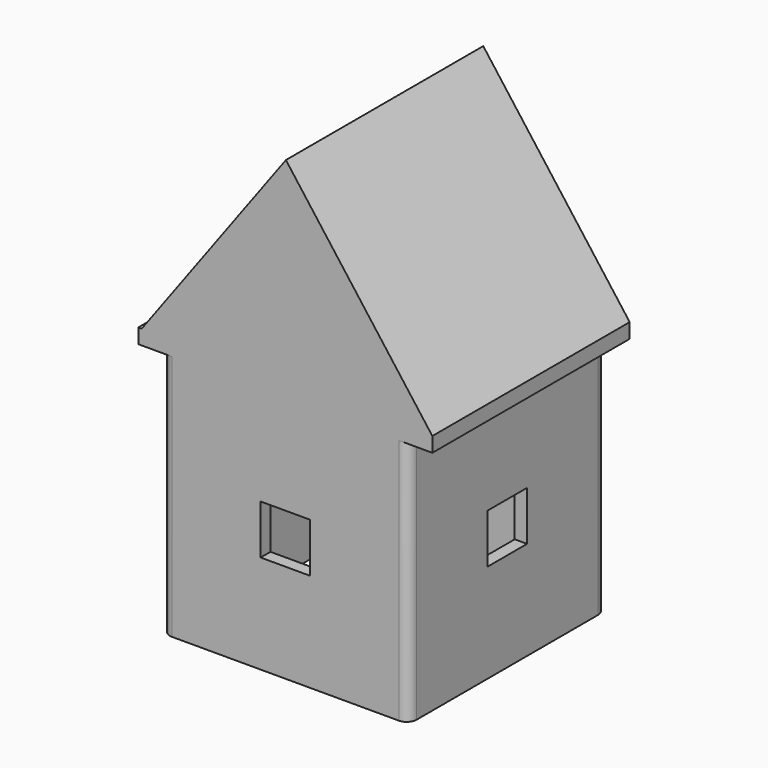
from build123d import *

# Parameters (mm, degrees)
F0_W      = 127
F0_H      = 127
F0_W_2    = 114.3
F0_H_2    = 114.3
F1_DEPTH  = 127
F2_W      = 25.4
F2_H      = 25.4
F3_DEPTH  = 6.35
F6_COUNT  = 4
F7_R      = 5.08
F9_DEPTH  = 7.62
F11_DEPTH = 127


with BuildPart() as f1:
    # F0 (on Top) → F1 (new body)
    with BuildSketch(Plane.XY):
        with Locations((-0.4615932703, 33.8642211668)):
            Rectangle(F0_W, F0_H)
        with Locations((-0.4615932703, 33.8642211668)):
            Rectangle(F0_W_2, F0_H_2, mode=Mode.SUBTRACT)
    extrude(amount=F1_DEPTH)

    # F2 (on face) → F3 (cut, through all)
    with BuildSketch(Plane.YZ.offset(63.0384067297)):
        with Locations((33.8642211668, 63.5)):
            Rectangle(F2_W, F2_H)
    f3 = extrude(amount=-F3_DEPTH, mode=Mode.SUBTRACT)

    # F6: F3 ×4 about axis
    f6_axis = Axis((-0.4615932703, 33.8642211668, 78.3742320016), (0, 0, -1))
    for i in range(1, F6_COUNT):
        add(f3.rotate(f6_axis, i * 360 / F6_COUNT), mode=Mode.SUBTRACT)

    # F7
    f7_edges = [f1.edges().sort_by_distance(p)[0] for p in [
        (-63.961593, -29.635779, 63.5),
        (63.038407, -29.635779, 63.5),
        (-63.961593, 97.364221, 63.5),
        (56.688407, 91.014221, 63.5),
        (63.038407, 97.364221, 63.5),
        (-57.611593, 91.014221, 63.5),
        (-57.611593, -23.285779, 63.5),
        (56.688407, -23.285779, 63.5),
    ]]
    fillet(f7_edges, radius=F7_R)

    # F8 (on face) → F9 (join)
    with BuildSketch(Plane.XY.offset(127)):
        with BuildLine():
            ThreePointArc((63.0384067297, -24.5557788332), (61.5505091781, -28.1478812816), (57.9584067297, -29.6357788332))
            Line((57.9584067297, -29.6357788332), (75.2250626683, -29.6357788332))
            Line((75.2250626683, -29.6357788332), (75.2250626683, 97.3642211668))
            Line((75.2250626683, 97.3642211668), (57.9584067297, 97.3642211668))
            ThreePointArc((57.9584067297, 97.3642211668), (61.5505091781, 95.8763236152), (63.0384067297, 92.2842211668))
            Line((63.0384067297, 92.2842211668), (63.0384067297, -24.5557788332))
        make_face()
        with BuildLine():
            ThreePointArc((-63.9615932703, -24.5557788332), (-62.4736957187, -28.1478812816), (-58.8815932703, -29.6357788332))
            Line((-58.8815932703, -29.6357788332), (57.9584067297, -29.6357788332))
            ThreePointArc((57.9584067297, -29.6357788332), (61.5505091781, -28.1478812816), (63.0384067297, -24.5557788332))
            Line((63.0384067297, -24.5557788332), (63.0384067297, 92.2842211668))
            ThreePointArc((63.0384067297, 92.2842211668), (61.5505091781, 95.8763236152), (57.9584067297, 97.3642211668))
            Line((57.9584067297, 97.3642211668), (-58.8815932703, 97.3642211668))
            ThreePointArc((-58.8815932703, 97.3642211668), (-62.4736957187, 95.8763236152), (-63.9615932703, 92.2842211668))
            Line((-63.9615932703, 92.2842211668), (-63.9615932703, -24.5557788332))
        make_face()
        with BuildLine():
            ThreePointArc((-52.5315932703, -23.2857788332), (-56.1236957187, -21.7978812816), (-57.6115932703, -18.2057788332))
            Line((-57.6115932703, -18.2057788332), (-57.6115932703, 85.9342211668))
            ThreePointArc((-57.6115932703, 85.9342211668), (-56.1236957187, 89.5263236152), (-52.5315932703, 91.0142211668))
            Line((-52.5315932703, 91.0142211668), (51.6084067297, 91.0142211668))
            ThreePointArc((51.6084067297, 91.0142211668), (55.2005091781, 89.5263236152), (56.6884067297, 85.9342211668))
            Line((56.6884067297, 85.9342211668), (56.6884067297, -18.2057788332))
            ThreePointArc((56.6884067297, -18.2057788332), (55.2005091781, -21.7978812816), (51.6084067297, -23.2857788332))
            Line((51.6084067297, -23.2857788332), (-52.5315932703, -23.2857788332))
        make_face(mode=Mode.SUBTRACT)
        with BuildLine():
            Line((-57.6115932703, 85.9342211668), (-57.6115932703, -18.2057788332))
            ThreePointArc((-57.6115932703, -18.2057788332), (-56.1236957187, -21.7978812816), (-52.5315932703, -23.2857788332))
            Line((-52.5315932703, -23.2857788332), (51.6084067297, -23.2857788332))
            ThreePointArc((51.6084067297, -23.2857788332), (55.2005091781, -21.7978812816), (56.6884067297, -18.2057788332))
            Line((56.6884067297, -18.2057788332), (56.6884067297, 85.9342211668))
            ThreePointArc((56.6884067297, 85.9342211668), (55.2005091781, 89.5263236152), (51.6084067297, 91.0142211668))
            Line((51.6084067297, 91.0142211668), (-52.5315932703, 91.0142211668))
            ThreePointArc((-52.5315932703, 91.0142211668), (-56.1236957187, 89.5263236152), (-57.6115932703, 85.9342211668))
        make_face()
        with BuildLine():
            Line((-74.7978676376, 97.3642211668), (-76.1525549474, -29.6357788332))
            Line((-76.1525549474, -29.6357788332), (-58.8815932703, -29.6357788332))
            ThreePointArc((-58.8815932703, -29.6357788332), (-62.4736957187, -28.1478812816), (-63.9615932703, -24.5557788332))
            Line((-63.9615932703, -24.5557788332), (-63.9615932703, 92.2842211668))
            ThreePointArc((-63.9615932703, 92.2842211668), (-62.4736957187, 95.8763236152), (-58.8815932703, 97.3642211668))
            Line((-58.8815932703, 97.3642211668), (-74.7978676376, 97.3642211668))
        make_face()
    extrude(amount=F9_DEPTH)

    # F10 (on face) → F11 (join, through all)
    with BuildSketch(Plane(origin=(0, 97.3642211668, 0), x_dir=(-1, 0, 0), z_dir=(0, 1, 0))):
        Polygon((0.1627568882, 235.1974227433), (-75.2250626683, 134.62), (74.3815182296, 134.62), align=None)
    extrude(amount=-F11_DEPTH)


solid = f1.part
